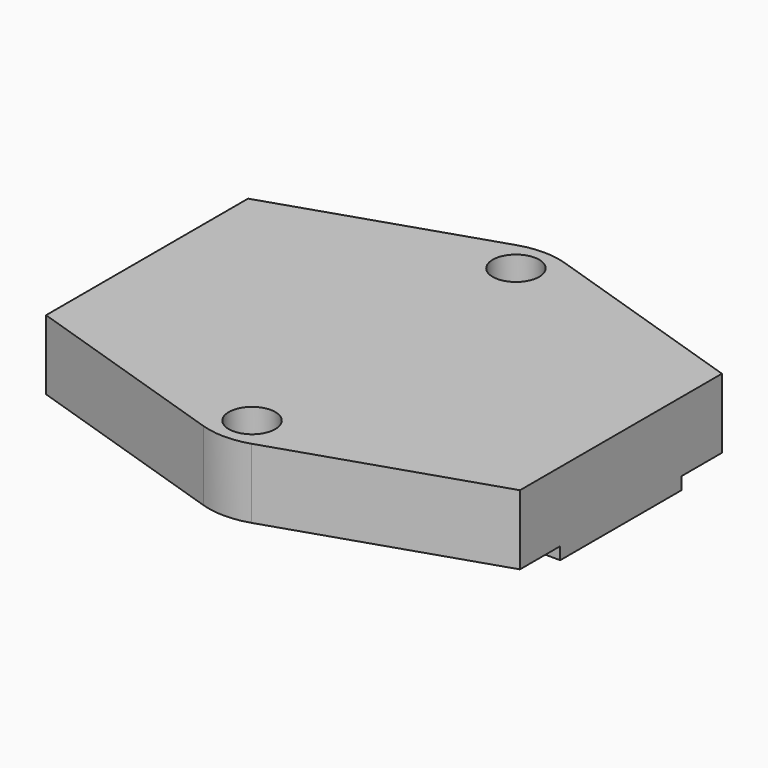
from build123d import *

# Parameters (mm, degrees)
F2_DEPTH = 1.6
F1_R     = 3
F1_W     = 3
F1_H     = 13.5
F1_H_2   = 11.6
F1_R_2   = 1.1303
F1_H_3   = 1.5
F3_DEPTH = 9
F4_DEPTH = 3
F5_DEPTH = 5
F6_DEPTH = 6.35
F7_R     = 3
F8_DEPTH = 3.5


with BuildPart() as f2:
    # F1 (on offset) → F2 (new body)
    with BuildSketch(Plane.XY.offset(18.75)):
        Polygon((28.1, -9.8), (30.6, -9.8), (30.6, 9.8), (28.1, 9.8), (28.1, 0), align=None)
    extrude(amount=-F2_DEPTH)

    # F1 (on offset) → F3 (join)
    with BuildSketch(Plane.XY.offset(18.75)):
        Polygon((-14.6, -13.3), (22.6, -13.3), (22.6, -10.3), (22.6, 10.3), (22.6, 13.3), (-14.6, 13.3), align=None)
        Polygon((-27.6, -13.3), (-14.6, -13.3), (-14.6, 13.3), (-27.6, 13.3), (-27.6, 1.7), (-27.6, -11.8), align=None)
        with BuildLine():
            Line((3.1063091707, -25.2848662841), (30.6, -16.3))
            Line((30.6, -16.3), (-30.6, -16.3))
            Line((-30.6, -16.3), (-3.1063091707, -25.2848662841))
            ThreePointArc((-3.1063091707, -25.2848662841), (0, -25.7795602219), (3.1063091707, -25.2848662841))
        make_face()
        with Locations((0, -21.3)):
            Circle(F1_R, mode=Mode.SUBTRACT)
        with BuildLine():
            Line((-30.6, 16.3), (30.6, 16.3))
            Line((30.6, 16.3), (3.1063091707, 25.2848662841))
            ThreePointArc((3.1063091707, 25.2848662841), (0, 25.7795602219), (-3.1063091707, 25.2848662841))
            Line((-3.1063091707, 25.2848662841), (-30.6, 16.3))
        make_face()
        with Locations((0, 21.3)):
            Circle(F1_R, mode=Mode.SUBTRACT)
        Polygon((27.6, -10.3), (27.6, -13.3), (22.6, -13.3), (-14.6, -13.3), (-27.6, -13.3), (-30.6, -13.3), (-30.6, -16.3), (30.6, -16.3), (30.6, -10.3), align=None)
        Polygon((27.6, 13.3), (27.6, 10.3), (30.6, 10.3), (30.6, 16.3), (-30.6, 16.3), (-30.6, 13.3), (-27.6, 13.3), (-14.6, 13.3), (22.6, 13.3), align=None)
        Polygon((22.6, -13.3), (27.6, -13.3), (27.6, -10.3), (27.6, 10.3), (27.6, 13.3), (22.6, 13.3), (22.6, 10.3), (22.6, -10.3), align=None)
        Polygon((28.1, -9.8), (30.6, -9.8), (30.6, 9.8), (28.1, 9.8), (28.1, 0), align=None)
        with Locations((-29.1, -5.05)):
            Rectangle(F1_W, F1_H)
        with Locations((-29.1, 7.5)):
            Rectangle(F1_W, F1_H_2)
        with Locations((0, 21.3)):
            Circle(F1_R)
        with Locations((0, 21.3)):
            Circle(F1_R_2, mode=Mode.SUBTRACT)
        with Locations((0, -21.3)):
            Circle(F1_R)
        with Locations((0, -21.3)):
            Circle(F1_R_2, mode=Mode.SUBTRACT)
        Polygon((27.6, 10.3), (27.6, -10.3), (30.6, -10.3), (30.6, -9.8), (28.1, -9.8), (28.1, 0), (28.1, 9.8), (30.6, 9.8), (30.6, 10.3), align=None)
        with Locations((-29.1, -12.55)):
            Rectangle(F1_W, F1_H_3)
        with Locations((0, -21.3)):
            Circle(F1_R_2)
    extrude(amount=F3_DEPTH)

    # F1 (on offset) → F4 (cut)
    with BuildSketch(Plane.XY.offset(18.75)):
        Polygon((-14.6, -13.3), (22.6, -13.3), (22.6, -10.3), (22.6, 10.3), (22.6, 13.3), (-14.6, 13.3), align=None)
        with Locations((0, -21.3)):
            Circle(F1_R_2)
    extrude(amount=F4_DEPTH, mode=Mode.SUBTRACT)

    # F1 (on offset) → F5 (cut)
    with BuildSketch(Plane.XY.offset(18.75)):
        with Locations((-29.1, -5.05)):
            Rectangle(F1_W, F1_H)
        with Locations((0, -21.3)):
            Circle(F1_R_2)
    extrude(amount=F5_DEPTH, mode=Mode.SUBTRACT)

    # F1 (on offset) → F6 (cut)
    with BuildSketch(Plane.XY.offset(18.75)):
        Polygon((-27.6, -13.3), (-14.6, -13.3), (-14.6, 13.3), (-27.6, 13.3), (-27.6, 1.7), (-27.6, -11.8), align=None)
        with Locations((0, -21.3)):
            Circle(F1_R_2)
    extrude(amount=F6_DEPTH, mode=Mode.SUBTRACT)

    # F7 (on face) → F8 (cut)
    with BuildSketch(Plane.XY.offset(27.75)):
        with Locations((0, 21.3)):
            Circle(F7_R)
        with Locations((0, -21.3)):
            Circle(F7_R)
    extrude(amount=-F8_DEPTH, mode=Mode.SUBTRACT)


solid = f2.part
